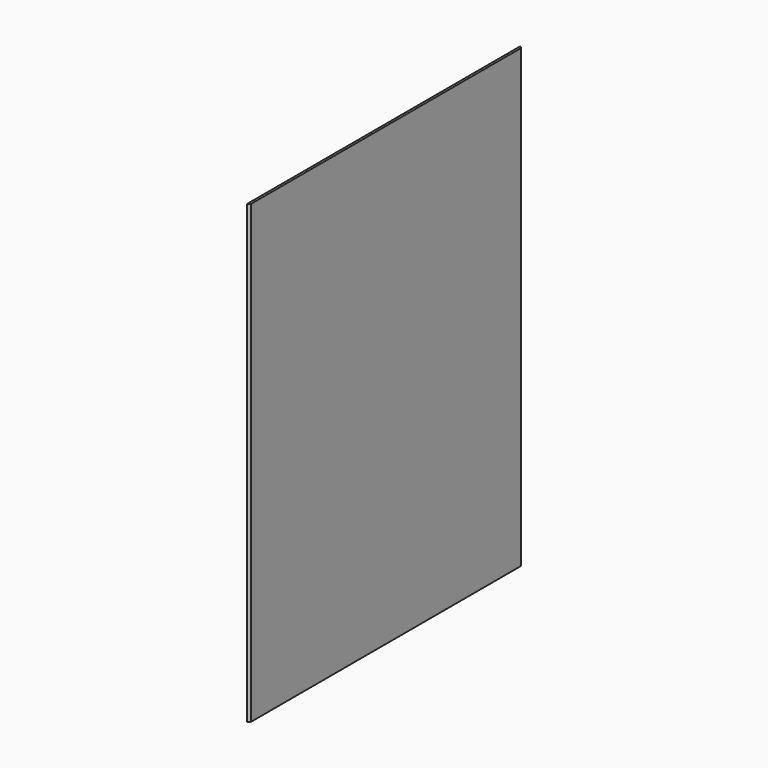
from build123d import *

# Parameters (mm, degrees)
F0_W     = 914.4
F0_H     = 1219.2
F1_DEPTH = 6.35
F2_SIZE  = 6.34999
F3_SIZE  = 6.34999


# Not quite as in the source:
# - a fillet or chamfer is up to 0.001 mm smaller than in the source, because OpenCascade refuses the exact size


with BuildPart() as f1:
    # F0 (on Right) → F1 (new body)
    with BuildSketch(Plane.YZ):
        Rectangle(F0_W, F0_H)
    extrude(amount=F1_DEPTH)

    # F2 (size 6.35 in the source; OpenCascade refuses exactly that, so slightly less here)
    f2_edges = [f1.edges().sort_by_distance(p)[0] for p in [
        (6.35, 457.2, 0),
    ]]
    chamfer(f2_edges, length=F2_SIZE)

    # F3 (size 6.35 in the source; OpenCascade refuses exactly that, so slightly less here)
    f3_edges = [f1.edges().sort_by_distance(p)[0] for p in [
        (6.35, -457.2, 0),
    ]]
    chamfer(f3_edges, length=F3_SIZE)


solid = f1.part
